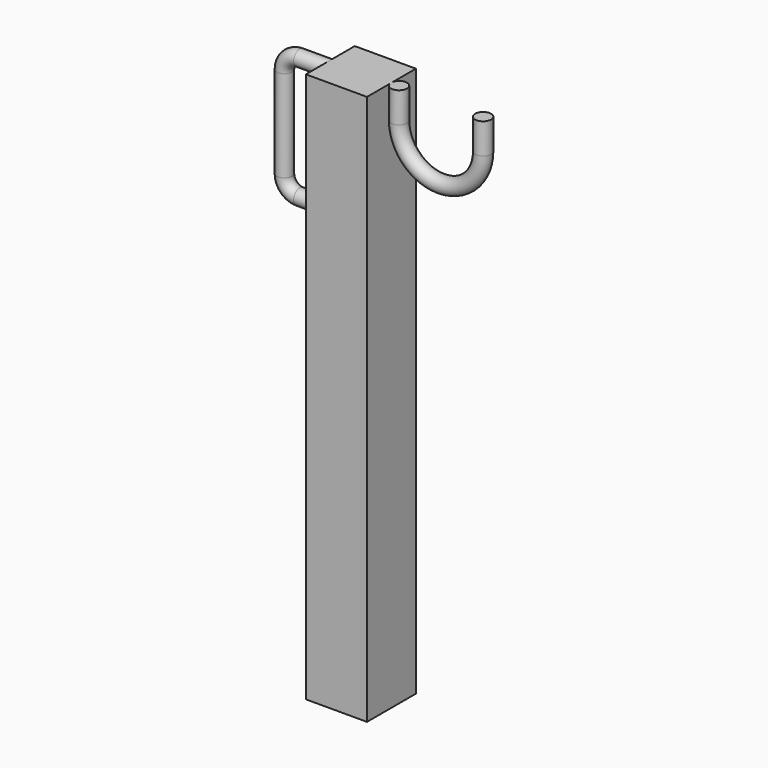
from build123d import *

# Parameters (mm, degrees)
F0_W          = 50.8
F0_H          = 50.8
F1_DEPTH      = 203.2
F1_DEPTH_BACK = 254
F3_R          = 6.604
F6_R          = 6.35


with BuildPart() as f1:
    # F0 (on Top) → F1 (new body, two sides)
    with BuildSketch(Plane.XY) as f1_sk:
        Rectangle(F0_W, F0_H)
    extrude(amount=F1_DEPTH)
    extrude(f1_sk.sketch, amount=-F1_DEPTH_BACK)

    # F4: sweep along a path in F2
    with BuildLine(Plane.XZ) as f4_path:
        Line((101.6, 203.2), (101.6, 177.8))
        ThreePointArc((101.6, 177.8), (66.675, 142.875), (31.75, 177.8))
        Line((31.75, 177.8), (31.75, 203.2))
    # F3 (on face) → F4 (sweep)
    with BuildSketch(Plane.XY.offset(203.2)):
        with Locations((31.75, 0)):
            Circle(F3_R)
    sweep(path=f4_path.line)

    # F7: sweep along a path in F5
    with BuildLine(Plane.XZ) as f7_path:
        Line((-25.4, 196.85), (-50.8, 196.85))
        ThreePointArc((-50.8, 196.85), (-59.7802561211, 193.1302561211), (-63.5, 184.15))
        Line((-63.5, 184.15), (-63.5, 107.95))
        ThreePointArc((-63.5, 107.95), (-59.7802561211, 98.9697438789), (-50.8, 95.25))
        Line((-50.8, 95.25), (-25.3296792507, 95.25))
    # F6 (on face) → F7 (sweep)
    with BuildSketch(Plane(origin=(-25.4, 0, 0), x_dir=(0, -1, 0), z_dir=(-1, 0, 0))):
        with Locations((0, 196.85)):
            Circle(F6_R)
    sweep(path=f7_path.line)


solid = f1.part
